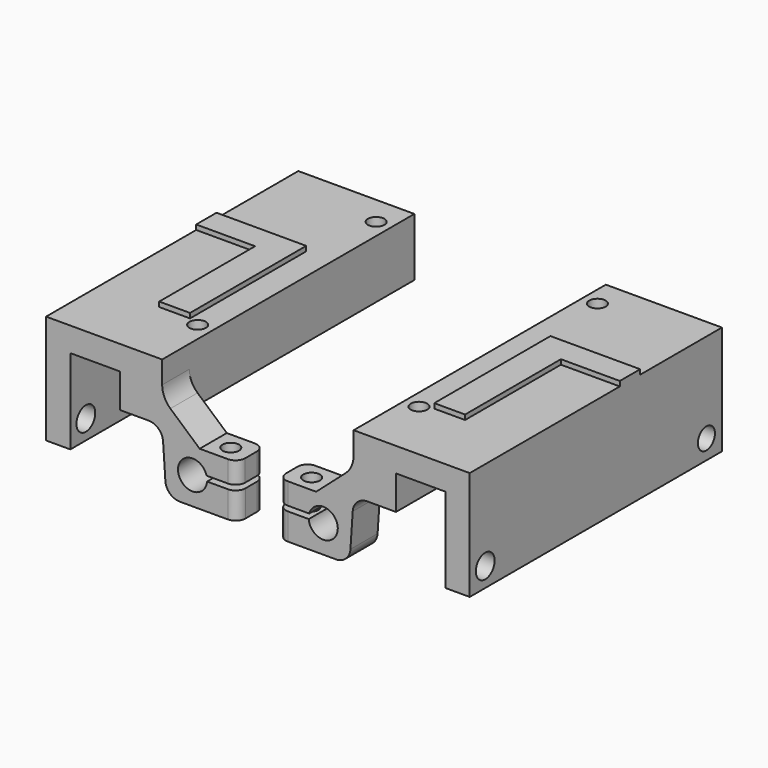
from build123d import *

# Parameters (mm, degrees)
F1_DEPTH      = 7
F2_DEPTH      = 58
F3_R          = 1.7
F3_R_2        = 11
F4_DEPTH      = 12.001
F5_R          = 3
F6_DEPTH      = 10
F7_DEPTH      = 12.001
F8_R          = 1.4
F9_DEPTH      = 10.9458027797
F8_R_2        = 1.7
F10_DEPTH     = 4.4233228002
F11_R         = 5
F12_R         = 3
F13_R         = 3
F14_R         = 2
F15_R         = 2.2
F15_R_2       = 2.4255023423
F16_DEPTH     = 6
F17_TEXT_SIZE = 41.9437823343
F18_DEPTH     = 1


# Not quite as in the source:
# - a feature names something its author has since deleted; it is built from what else it names
# - Text() gives the source's letters only with a copy of the font that has no kerning and outlines rounded to 1/6400 em; it was checked with that copy


with BuildPart() as f1:
    # F0 (on Front) → F1 (new body)
    with BuildSketch(Plane.XZ):
        Polygon((-18.6721007523, 29.8099789735), (-18.6721007523, 7.3259699669), (-13.6721007523, 7.3259699669), (-13.6721007523, 24.8099789735), (-3.4721007523, 24.8099789735), (-3.4721007523, 17.8099789735), (5.2637966118, 17.8099789735), (5.2637966118, 22.9406704692), (5.2637966118, 29.8099789735), align=None)
        Polygon((12.9923354834, 16.1279886961), (5.2637966118, 22.9406704692), (5.2637966118, 17.8099789735), (6.1103762127, 5.1831859164), (20.8186601057, 5.1831859164), (20.8186601057, 10.6682249423), (13.4860510706, 10.6682249423), (13.4860510706, 11.7046658959), (20.7896428882, 11.7046658959), (20.7896428882, 16.1279886961), align=None)
    extrude(amount=F1_DEPTH)

    # F0 (on Front) → F2 (join)
    with BuildSketch(Plane.XZ):
        Polygon((-18.6721007523, 29.8099789735), (-18.6721007523, 7.3259699669), (-13.6721007523, 7.3259699669), (-13.6721007523, 24.8099789735), (-3.4721007523, 24.8099789735), (-3.4721007523, 17.8099789735), (5.2637966118, 17.8099789735), (5.2637966118, 22.9406704692), (5.2637966118, 29.8099789735), align=None)
    extrude(amount=-F2_DEPTH)

    # F3 (on face) → F4 (cut, through all)
    with BuildSketch(Plane(origin=(0, 0, 17.8099789735), x_dir=(1, 0, 0), z_dir=(0, 0, -1))):
        with Locations((2.1850741468, -6)):
            Circle(F3_R)
        with Locations((2.1850741468, -52)):
            Circle(F3_R)
        with Locations((17.6850741468, -29)):
            Circle(F3_R_2)
    extrude(amount=-F4_DEPTH, mode=Mode.SUBTRACT)

    # F5 (on face) → F6 (cut)
    with BuildSketch(Plane.XZ.offset(7)):
        with Locations((11.5278992477, 10.8989789735)):
            Circle(F5_R)
    extrude(amount=-F6_DEPTH, mode=Mode.SUBTRACT)

    # F3 (on face) → F7 (cut, through all)
    with BuildSketch(Plane(origin=(0, 0, 17.8099789735), x_dir=(1, 0, 0), z_dir=(0, 0, -1))):
        with Locations((2.1850741468, -6)):
            Circle(F3_R)
        with Locations((2.1850741468, -52)):
            Circle(F3_R)
        with Locations((17.6850741468, -29)):
            Circle(F3_R_2)
    extrude(amount=-F7_DEPTH, mode=Mode.SUBTRACT)

    # F8 (on face) → F9 (cut, through all)
    with BuildSketch(Plane.XY.offset(16.1279886961)):
        with Locations((16.669401899, -3.5767070949)):
            Circle(F8_R)
    extrude(amount=-F9_DEPTH, mode=Mode.SUBTRACT)

    # F8 (on face) → F10 (cut, through all)
    with BuildSketch(Plane.XY.offset(16.1279886961)):
        with Locations((16.669401899, -3.5767070949)):
            Circle(F8_R_2)
        with Locations((16.669401899, -3.5767070949)):
            Circle(F8_R, mode=Mode.SUBTRACT)
    extrude(amount=-F10_DEPTH, mode=Mode.SUBTRACT)

    # F11
    f11_edges = [f1.edges().sort_by_distance(p)[0] for p in [
        (5.263797, -3.5, 22.94067),
    ]]
    fillet(f11_edges, radius=F11_R)

    # F12
    f12_edges = [f1.edges().sort_by_distance(p)[0] for p in [
        (5.263797, -3.5, 17.809979),
    ]]
    fillet(f12_edges, radius=F12_R)

    # F13
    f13_edges = [f1.edges().sort_by_distance(p)[0] for p in [
        (6.110376, -3.5, 5.183186),
    ]]
    fillet(f13_edges, radius=F13_R)

    # F14
    f14_edges = [f1.edges().sort_by_distance(p)[0] for p in [
        (20.789643, -7, 13.916327),
        (20.81866, -7, 7.925705),
        (20.789643, 0, 13.916327),
        (20.81866, 0, 7.925705),
    ]]
    fillet(f14_edges, radius=F14_R)

    # F15 (on face) → F16 (cut)
    with BuildSketch(Plane(origin=(-18.6721007523, 0, 0), x_dir=(0, -1, 0), z_dir=(-1, 0, 0))):
        with Locations((-54, 11.3259699669)):
            Circle(F15_R)
        with Locations((3, 11.3259699669)):
            Circle(F15_R_2)
    extrude(amount=-F16_DEPTH, mode=Mode.SUBTRACT)

    # F17 (on face) → F18 (join)
    with BuildSketch(Plane.XY.offset(29.8099789735)):
        with Locations(Location((3.5908724648, 36.9253193088), (0, 0, 180))):
            Text('L', F17_TEXT_SIZE, font='Open Sans', font_style=FontStyle.BOLD, text_align=(TextAlign.LEFT, TextAlign.BOTTOM))
    extrude(amount=F18_DEPTH)


with BuildPart() as f19_1:
    # F19: instance of F1
    add(f1.part.mirror(Plane.YZ))


with BuildPart() as f19_1_1:
    # F20: moved
    add(f19_1.part.moved(Location((50, 0, 0))))


solid = Compound([f1.part, f19_1_1.part])
